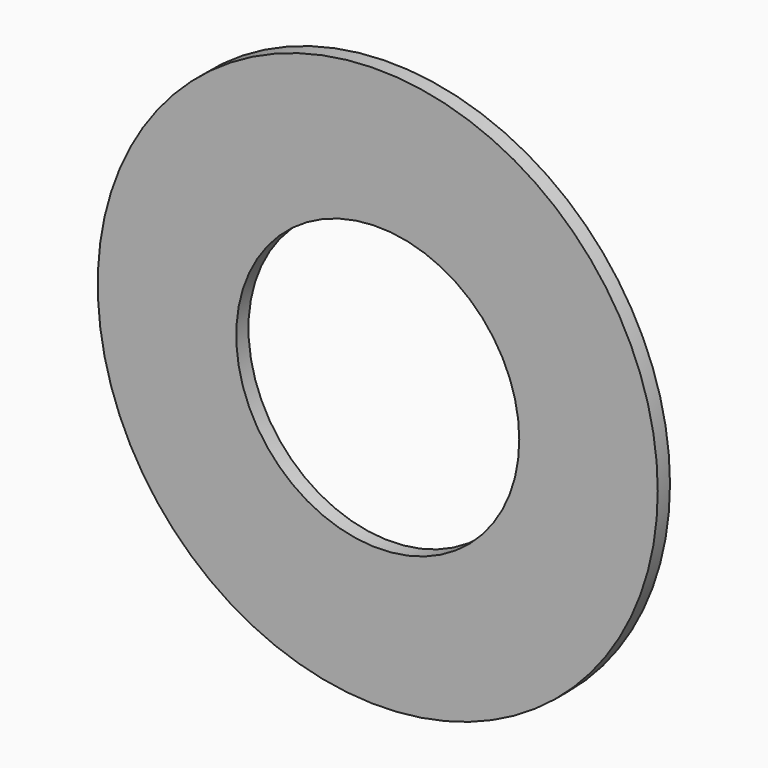
from build123d import *

# Parameters (mm, degrees)
F0_R     = 91.60262799
F0_R_2   = 57.3129322619
F0_R_3   = 46.2963533707
F1_DEPTH = 5


# Not quite as in the source:
# - the program builds the solid bodies; features that only make, move or delete a surface that nothing else refers to are left out


with BuildPart() as f1:
    # F0 (on Front) → F1 (new body)
    with BuildSketch(Plane.XZ):
        Circle(F0_R)
        Circle(F0_R_2, mode=Mode.SUBTRACT)
        Circle(F0_R_2)
        Circle(F0_R_3, mode=Mode.SUBTRACT)
    extrude(amount=F1_DEPTH)


solid = f1.part
